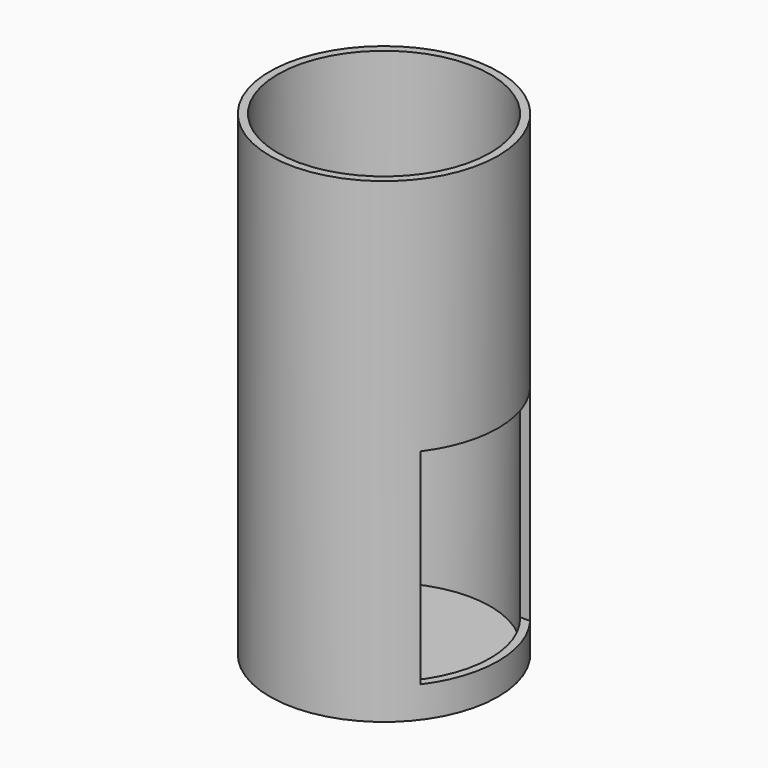
from build123d import *

# Parameters (mm, degrees)
F0_R     = 35.9798684942
F1_DEPTH = 150
F2_T     = -2.5
F4_W     = 21.6136686504
F4_H     = 64.6223351359
F5_DEPTH = 150


with BuildPart() as f1:
    # F0 (on Top) → F1 (new body)
    with BuildSketch(Plane.XY):
        Circle(F0_R)
    extrude(amount=F1_DEPTH)

    # F2
    f2_openings = [f1.faces().sort_by_distance(p)[0] for p in [
        (0, 0, 150),
    ]]
    offset(amount=F2_T, openings=f2_openings)

    # F4 (on face) → F5 (cut)
    with BuildSketch(Plane(origin=(35.9798684942, 0, 0), x_dir=(0, -1, 0), z_dir=(-1, 0, 0))):
        with Locations((10.8068343252, 42.1714968979)):
            Rectangle(F4_W, F4_H)
        with Locations((-10.8068343252, 42.1714968979)):
            Rectangle(F4_W, F4_H)
    extrude(amount=F5_DEPTH, mode=Mode.SUBTRACT)


solid = f1.part
